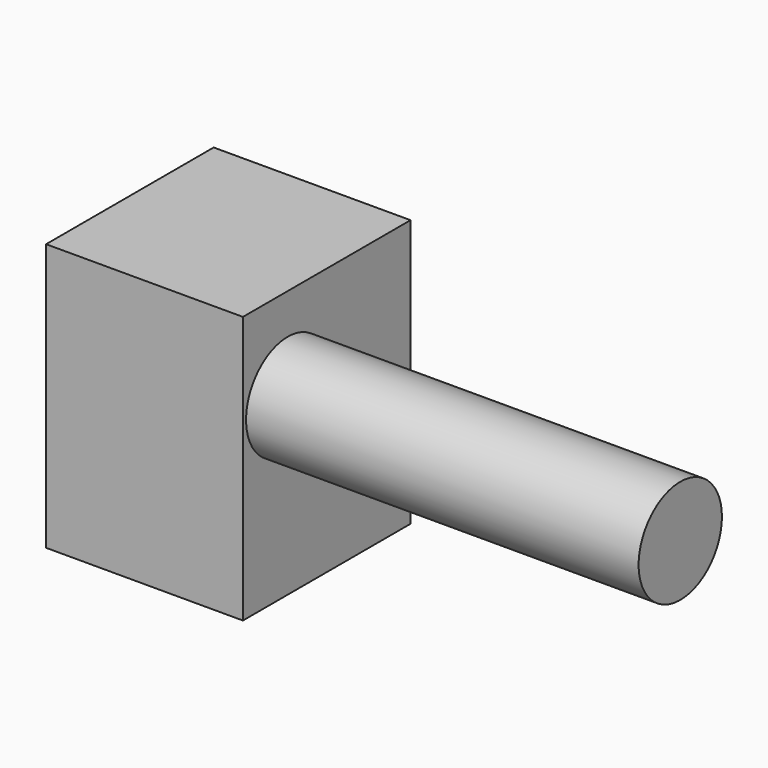
from build123d import *

# Parameters (mm, degrees)
F0_W          = 93.5181863606
F0_H          = 99.5218157768
F1_DEPTH      = 127
F2_R          = 24.7334517627
F3_DEPTH      = 186.5019382
F3_DEPTH_BACK = 41.98141


# Not quite as in the source:
# - an extrude ends at something that could not be found from the text; its depth is read off the source's solid


with BuildPart() as f1:
    # F0 (on Top) → F1 (new body)
    with BuildSketch(Plane.XY):
        with Locations((3.8100015372, -1.3854540884)):
            Rectangle(F0_W, F0_H)
    extrude(amount=F1_DEPTH)

    # F2 (on face) → F3 (join, two sides)
    with BuildSketch(Plane.YZ.offset(50.5690947175)) as f3_sk:
        with Locations((-24.546951997, 83.1744330844)):
            Circle(F2_R)
    extrude(amount=F3_DEPTH)
    extrude(f3_sk.sketch, amount=-F3_DEPTH_BACK)


solid = f1.part
